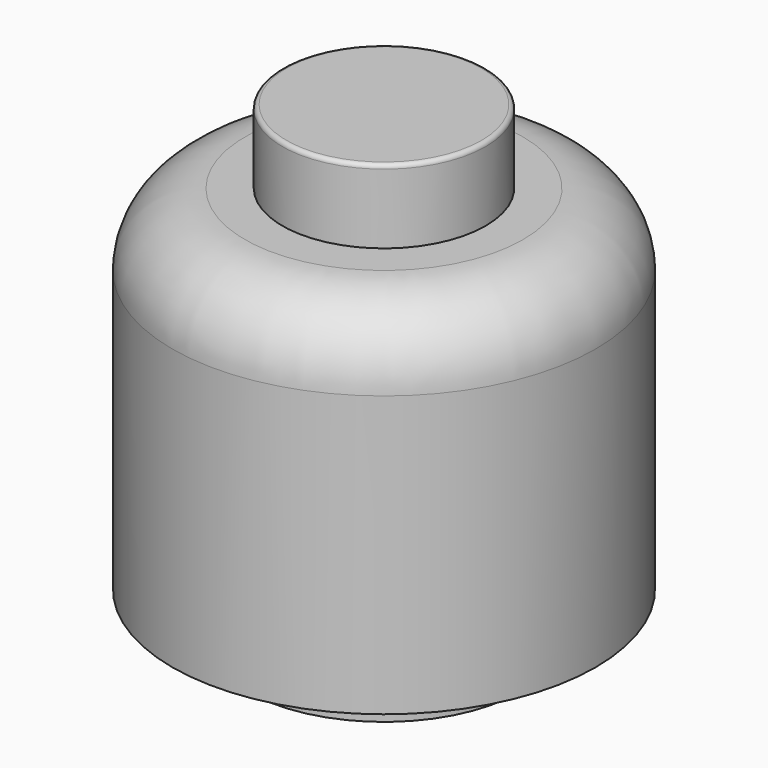
from build123d import *

# Parameters (mm, degrees)
F0_R     = 51
F1_DEPTH = 42.5
F2_R     = 17.5
F3_R     = 24.5
F4_DEPTH = 17.8
F5_R     = 1
F6_DEPTH = 42.5
F7_R     = 33
F8_DEPTH = 11


# Not quite as in the source:
# - a feature of the source that left no trace in its solid (it failed there, or was rolled back) is left out


with BuildPart() as f1:
    # F0 (on Top) → F1 (new body)
    with BuildSketch(Plane.XY):
        Circle(F0_R)
    extrude(amount=F1_DEPTH)

    # F2
    f2_edges = [f1.edges().sort_by_distance(p)[0] for p in [
        (-51, 0, 42.5),
    ]]
    fillet(f2_edges, radius=F2_R)

    # F3 (on face) → F4 (join)
    with BuildSketch(Plane.XY.offset(42.5)):
        Circle(F3_R)
    extrude(amount=F4_DEPTH)

    # F5
    f5_edges = [f1.edges().sort_by_distance(p)[0] for p in [
        (-24.5, 0, 60.3),
    ]]
    fillet(f5_edges, radius=F5_R)

    # F6 (add): a face of the model
    f6_faces = [f1.faces().sort_by_distance(p)[0] for p in [
        (0, 0, 0),
    ]]
    extrude(f6_faces, amount=F6_DEPTH)

    # F7 (on face) → F8 (join)
    with BuildSketch(Plane(origin=(0, 0, -42.5), x_dir=(1, 0, 0), z_dir=(0, 0, -1))):
        Circle(F7_R)
    extrude(amount=F8_DEPTH)


solid = f1.part
